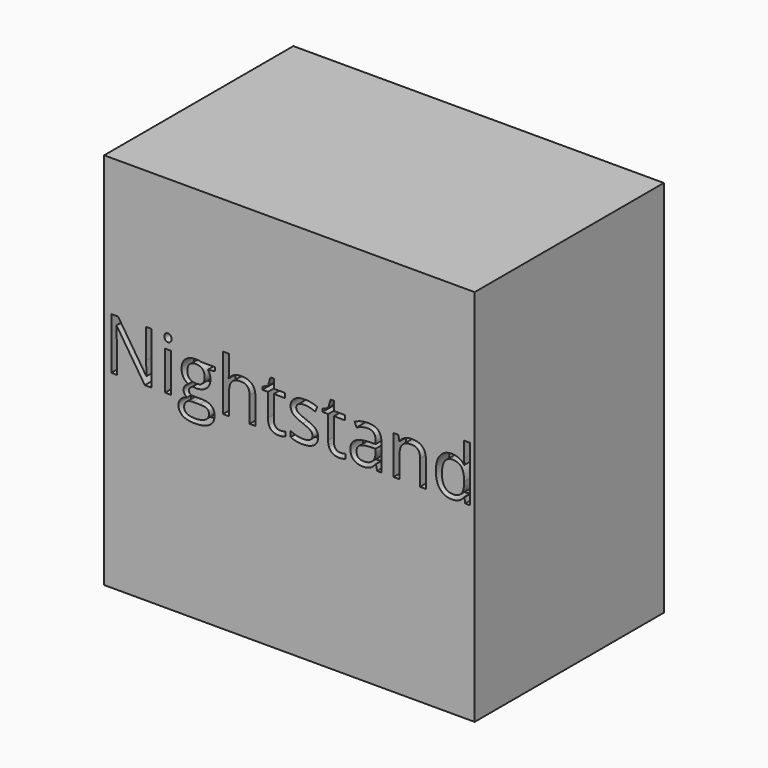
from build123d import *

# Parameters (mm, degrees)
F0_W         = 596.9
F0_H         = 609.6
F1_DEPTH     = 190.5
F2_TEXT_SIZE = 116.7423524738
F3_DEPTH     = 25.4


# Not quite as in the source:
# - Text() gives the source's letters only with a copy of the font that has no kerning and outlines rounded to 1/6400 em; it was checked with that copy


with BuildPart() as f1:
    # F0 (on Front) → F1 (new body, symmetric)
    with BuildSketch(Plane.XZ):
        Rectangle(F0_W, F0_H)
    extrude(amount=F1_DEPTH, both=True)

    # F2 (on face) → F3 (cut)
    with BuildSketch(Plane.XZ.offset(190.5)):
        with Locations((-298.45, 0)):
            Text('Nightstand', F2_TEXT_SIZE, font='Open Sans', text_align=(TextAlign.LEFT, TextAlign.BOTTOM))
    extrude(amount=-F3_DEPTH, mode=Mode.SUBTRACT)


solid = f1.part
